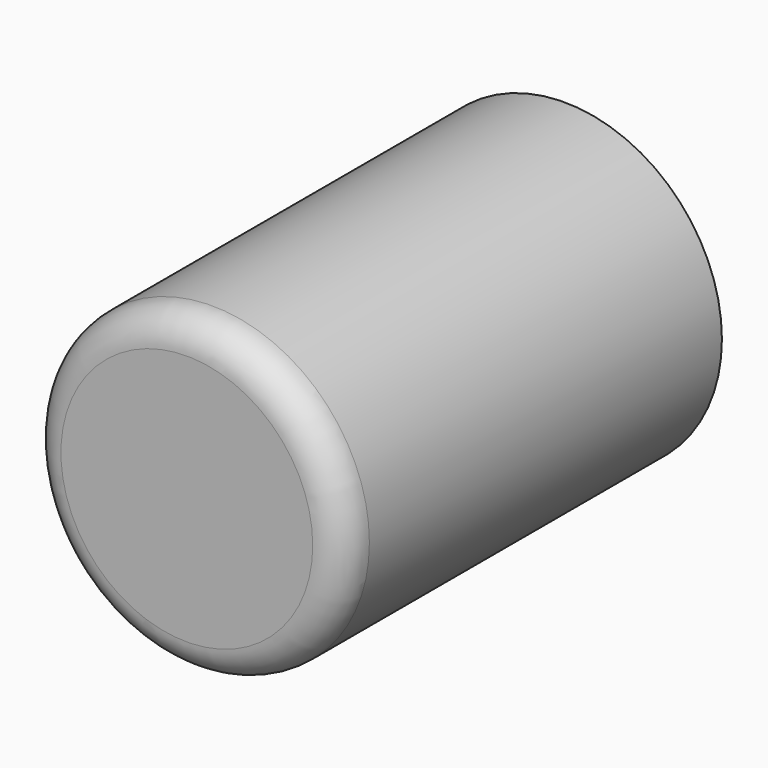
from build123d import *

# Parameters (mm, degrees)
F2_R     = 10
F1_R     = 10
F4_R     = 2
F6_DEPTH = 25


with BuildPart() as f3:
    # F2 (on Front) → F3 section 0
    with BuildSketch(Plane.XZ):
        Circle(F2_R)
    # F1 (on offset) → F3 section 1
    with BuildSketch(Plane.XZ.offset(30)):
        Circle(F1_R)
    loft()

    # F4
    f4_edges = [f3.edges().sort_by_distance(p)[0] for p in [
        (-10, -30, 0),
    ]]
    fillet(f4_edges, radius=F4_R)

    # F5 (on Front) → F6 (cut)
    with BuildSketch(Plane.XZ):
        with BuildLine():
            ThreePointArc((-4.1235491527, 2.8277804697), (-1.4802456276, -4.7758635745), (5, 0))
            ThreePointArc((5, 0), (4.7758635745, 1.4802456276), (4.1235491527, 2.8277804697))
            Line((4.1235491527, 2.8277804697), (-4.1235491527, 2.8277804697))
        make_face()
    extrude(amount=F6_DEPTH, mode=Mode.SUBTRACT)


solid = f3.part
